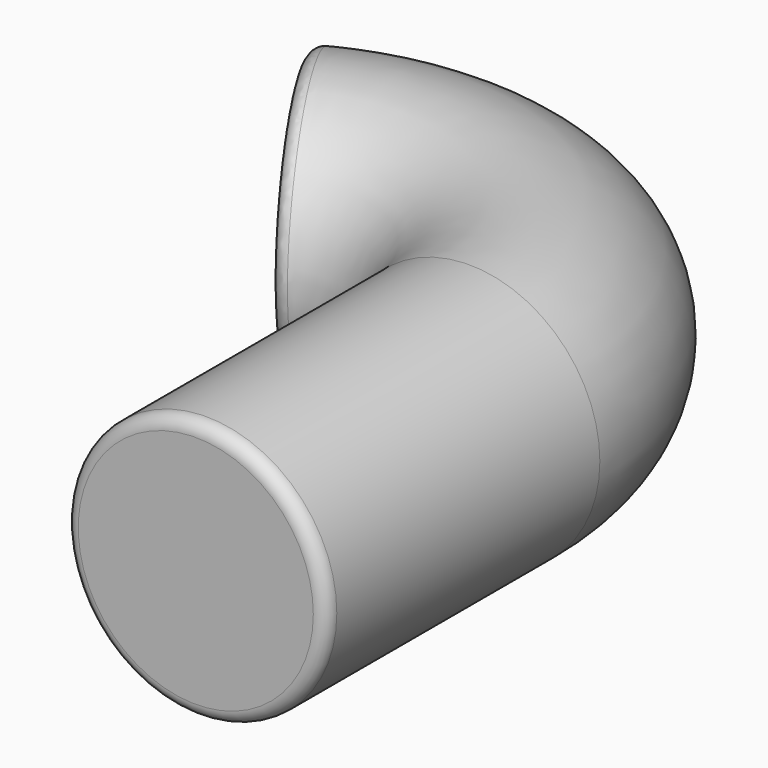
from build123d import *

# Parameters (mm, degrees)
F1_R      = 100
F2_FACE_R = 100
F4_R      = 158.537666862
F4_R_2    = 100
F5_DEPTH  = 261
F6_R      = 10
F7_R      = 10


with BuildPart() as f2:
    # F2: sweep along a path in F0
    with BuildLine(Plane.XY) as f2_path:
        ThreePointArc((161.8, 0), (80.7807923206, 140.1916673417), (-81.1382397041, 139.9850922696))
    # F1 (on Front) → F2 (sweep)
    with BuildSketch(Plane.XZ):
        with Locations((161.8, 0)):
            Circle(F1_R)
    sweep(path=f2_path.line)

    # F3: sweep along a path in F0
    with BuildLine(Plane.XY) as f3_path:
        Line((161.8, 0), (161.8, -261.8))
    # F2_face (on face) → F3 (sweep)
    with BuildSketch(Plane(origin=(161.8, 0, 0), x_dir=(1, 0, 0), z_dir=(0, -1, 0))):
        Circle(F2_FACE_R)
    sweep(path=f3_path.line)

    # F4 (on face) → F5 (cut)
    with BuildSketch(Plane.XZ.offset(261.8)):
        with Locations((161.8, 0)):
            Circle(F4_R)
        with Locations((161.8, 0)):
            Circle(F4_R_2, mode=Mode.SUBTRACT)
    extrude(amount=-F5_DEPTH, mode=Mode.SUBTRACT)

    # F6
    f6_edges = [f2.edges().sort_by_distance(p)[0] for p in [
        (61.8, 0, 0),
        (61.8, -261.8, 0),
        (261.8, -130.9, 0),
    ]]
    fillet(f6_edges, radius=F6_R)

    # F7
    f7_edges = [f2.edges().sort_by_distance(p)[0] for p in [
        (-30.990996, 53.46773, 0),
    ]]
    fillet(f7_edges, radius=F7_R)


solid = f2.part
